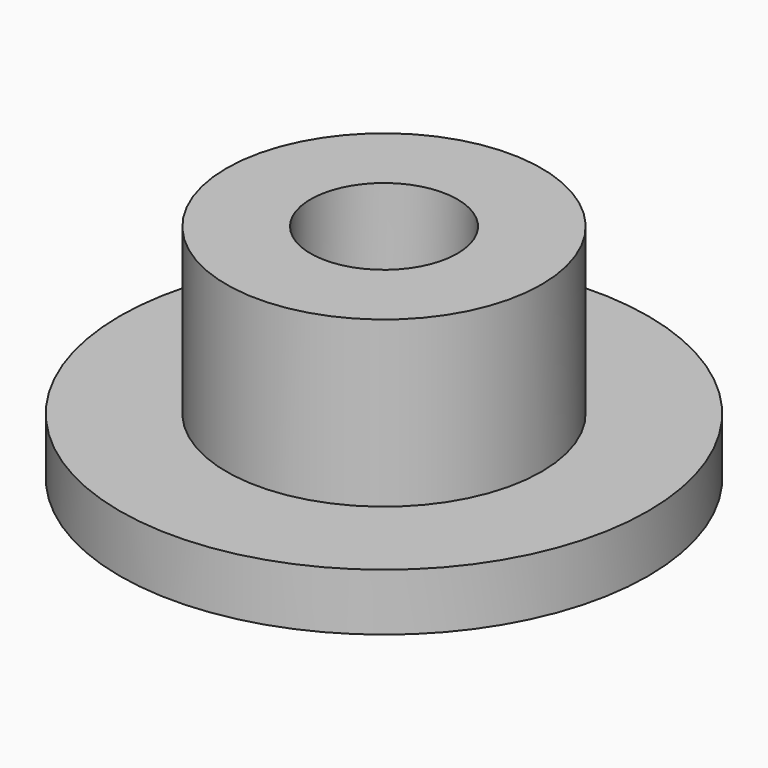
from build123d import *

# Parameters (mm, degrees)
F0_R     = 4.6841242686
F1_DEPTH = 4.9
F2_R     = 7.8548268631
F3_DEPTH = 1.7
F4_T     = 2.5


# Not quite as in the source:
# - a shell that OpenCascade refuses in one call is made with other operations: the cavity is built on its own and cut out


with BuildPart() as f1:
    # F0 (on Top) → F1 (new body)
    with BuildSketch(Plane.XY):
        Circle(F0_R)
    extrude(amount=F1_DEPTH)

    # F2 (on face) → F3 (join)
    with BuildSketch(Plane(origin=(0, 0, 0), x_dir=(1, 0, 0), z_dir=(0, 0, -1))):
        Circle(F2_R)
    extrude(amount=F3_DEPTH)

    # F4: shell of thickness 2.5, made by hand


with BuildPart() as f4_core1:
    # F4_t2: copy of F1
    add(f1.part)

    # the walls: a layer under each face that stays
    f4_faces = [f4_core1.faces().sort_by_distance(p)[0] for p in [
        (-7.8548268631, 0, -0.85),
        (0, 0, -1.7),
        (-4.6841242686, 0, 2.45),
    ]]
    thicken(f4_faces, amount=-F4_T, mode=Mode.SUBTRACT)


with BuildPart() as f1_1:
    add(f1.part)

    # what is left inside the walls is the cavity
    f4_cavity = [f4_core1.part.solids().sort_by_distance(p)[0] for p in [
        (-2.159124, 0, 3.533333),
    ]]
    add(f4_cavity, mode=Mode.SUBTRACT)


solid = f1_1.part
